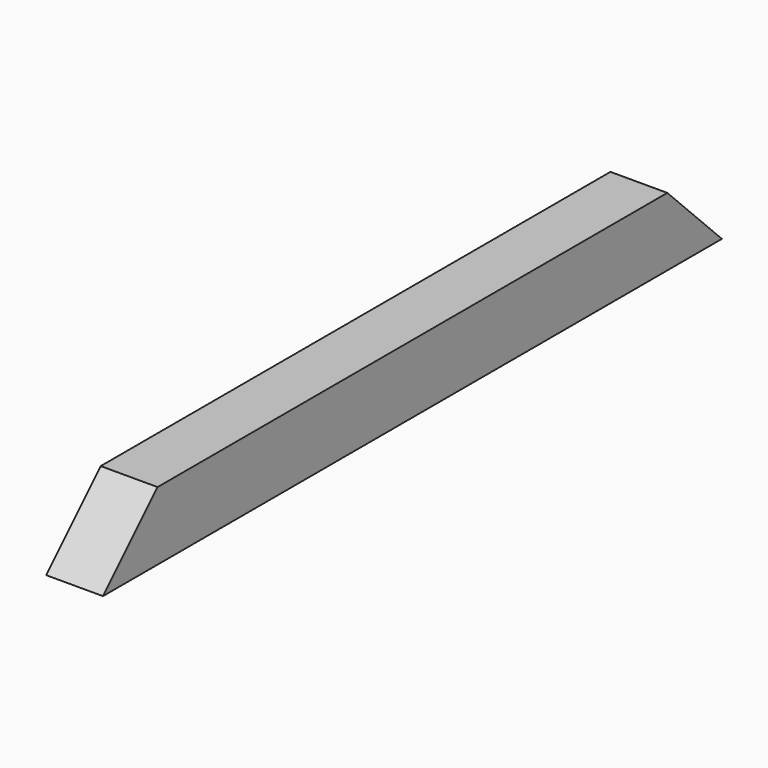
from build123d import *

# Parameters (mm, degrees)
F0_W     = 215.9
F0_H     = 19.05
F1_DEPTH = 7.9375
F2_SIZE2 = 19.04999
F2_SIZE  = 19.04999
F3_SIZE2 = 19.04999
F3_SIZE  = 19.04999


# Not quite as in the source:
# - a fillet or chamfer is up to 0.001 mm smaller than in the source, because OpenCascade refuses the exact size


with BuildPart() as f1:
    # F0 (on Right) → F1 (new body, symmetric)
    with BuildSketch(Plane.YZ):
        Rectangle(F0_W, F0_H)
    extrude(amount=F1_DEPTH, both=True)

    # F2 (size 19.05 and 19.05 in the source; OpenCascade refuses exactly that, so slightly less here)
    f2_edges = [f1.edges().sort_by_distance(p)[0] for p in [
        (0, -107.95, 9.525),
    ]]
    chamfer(f2_edges, length=F2_SIZE, length2=F2_SIZE2)

    # F3 (size 19.05 and 19.05 in the source; OpenCascade refuses exactly that, so slightly less here)
    f3_edges = [f1.edges().sort_by_distance(p)[0] for p in [
        (0, 107.95, 9.525),
    ]]
    chamfer(f3_edges, length=F3_SIZE, length2=F3_SIZE2)


solid = f1.part
